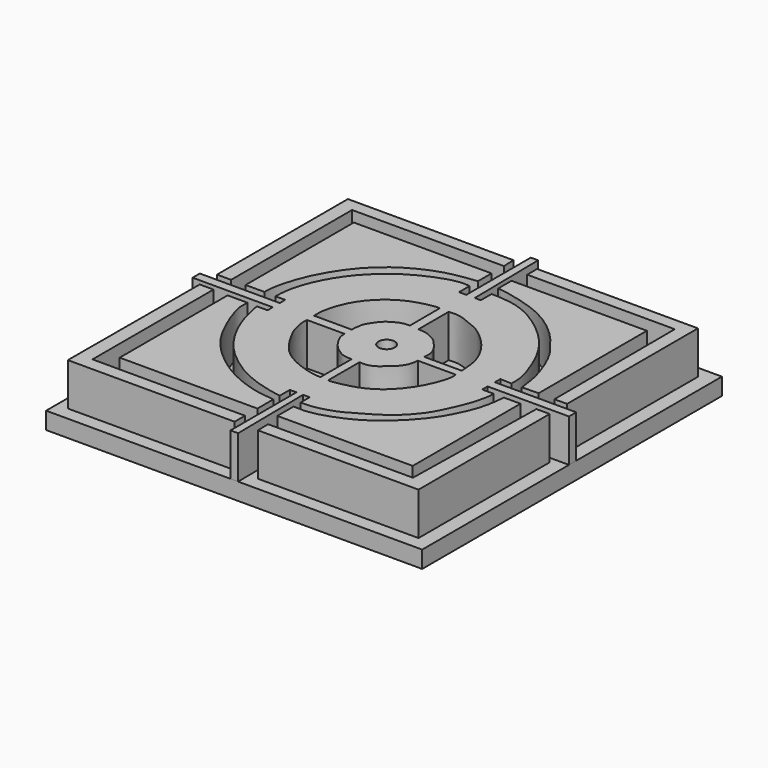
from build123d import *

# Parameters (mm, degrees)
F1_DEPTH = 5
F0_R     = 0.9585003227
F3_DEPTH = 2


# Not quite as in the source:
# - a feature names something its author has since deleted; it is built from what else it names


with BuildPart() as f1:
    # F0 (on Top) → F1 (new body)
    with BuildSketch(Plane.XY):
        with BuildLine():
            add(Edge.make_bspline(
                [(16.4221860468, 62.1270276606), (15.8832675467, 62.1270276606), (15.3443490465, 62.1270276606), (14.8054305464, 62.1270276606)],
                knots=[0, 0, 0, 0, 1.6167555004, 1.6167555004, 1.6167555004, 1.6167555004], degree=3))
            add(Edge.make_bspline(
                [(14.8054305464, 62.1270276606), (14.7858333463, 55.7044409215), (14.7662361463, 49.2818541825), (14.7466389462, 42.8592674434)],
                knots=[0, 0, 0, 0, 19.2678499122, 19.2678499122, 19.2678499122, 19.2678499122], degree=3))
            add(Edge.make_bspline(
                [(14.7466389462, 42.8592674434), (21.2821072588, 42.8592674434), (27.7793089098, 42.8592674434), (34.3147772225, 42.8592674434)],
                knots=[0, 0, 0, 0, 19.5681382762, 19.5681382762, 19.5681382762, 19.5681382762], degree=3))
            add(Edge.make_bspline(
                [(34.3147772225, 42.8592674434), (34.3147772225, 43.3677670856), (34.3147772225, 43.8762667278), (34.3147772225, 44.3847663701)],
                knots=[0, 0, 0, 0, 1.5254989266, 1.5254989266, 1.5254989266, 1.5254989266], degree=3))
            add(Edge.make_bspline(
                [(34.3147772225, 44.3847663701), (28.3378246101, 44.3847663701), (22.3991386592, 44.3847663701), (16.4221860468, 44.3847663701)],
                knots=[0, 0, 0, 0, 17.8925911756, 17.8925911756, 17.8925911756, 17.8925911756], degree=3))
            add(Edge.make_bspline(
                [(16.4221860468, 44.3847663701), (16.4221860468, 50.2988534669), (16.4221860468, 56.2129405638), (16.4221860468, 62.1270276606)],
                knots=[0, 0, 0, 0, 17.7422612906, 17.7422612906, 17.7422612906, 17.7422612906], degree=3))
        make_face()
    extrude(amount=-F1_DEPTH)


with BuildPart() as f1b:
    # F0 (on Top) → F1, piece 2 (new body)
    with BuildSketch(Plane.XY):
        with BuildLine():
            add(Edge.make_bspline(
                [(54.01673913, 44.3847663701), (48.3487062156, 44.3847663701), (42.6806733012, 44.3847663701), (37.0126403868, 44.3847663701)],
                knots=[0, 0, 0, 0, 17.0040987432, 17.0040987432, 17.0040987432, 17.0040987432], degree=3))
            add(Edge.make_bspline(
                [(37.0126403868, 44.3847663701), (37.0219697555, 43.8762667278), (37.0312991242, 43.3677670856), (37.0406284928, 42.8592674434)],
                knots=[0, 0, 0, 0, 1.5257556519, 1.5257556519, 1.5257556519, 1.5257556519], degree=3))
            add(Edge.make_bspline(
                [(37.0406284928, 42.8592674434), (43.3241464198, 42.8592674434), (49.6076643467, 42.8592674434), (55.8911822736, 42.8592674434)],
                knots=[0, 0, 0, 0, 18.8505537808, 18.8505537808, 18.8505537808, 18.8505537808], degree=3))
            add(Edge.make_bspline(
                [(55.8911822736, 42.8592674434), (55.8911822736, 49.2690689862), (55.8911822736, 55.6788705289), (55.8911822736, 62.0886720717)],
                knots=[0, 0, 0, 0, 19.2294046283, 19.2294046283, 19.2294046283, 19.2294046283], degree=3))
            add(Edge.make_bspline(
                [(55.8911822736, 62.0886720717), (55.3724678854, 62.0886720717), (54.8537534972, 62.0886720717), (54.335039109, 62.0886720717)],
                knots=[0, 0, 0, 0, 1.5561431646, 1.5561431646, 1.5561431646, 1.5561431646], degree=3))
            add(Edge.make_bspline(
                [(54.335039109, 62.0886720717), (54.228939116, 56.1873701711), (54.122839123, 50.2860682706), (54.01673913, 44.3847663701)],
                knots=[0, 0, 0, 0, 17.7067668412, 17.7067668412, 17.7067668412, 17.7067668412], degree=3))
        make_face()
    extrude(amount=-F1_DEPTH)


with BuildPart() as f1c:
    # F0 (on Top) → F1, piece 3 (new body)
    with BuildSketch(Plane.XY):
        with BuildLine():
            add(Edge.make_bspline(
                [(54.335039109, 82.3838636279), (54.3570650948, 76.470060481), (54.3790910807, 70.556257334), (54.4011170665, 64.6424541871)],
                knots=[0, 0, 0, 0, 17.7415324942, 17.7415324942, 17.7415324942, 17.7415324942], degree=3))
            add(Edge.make_bspline(
                [(54.4011170665, 64.6424541871), (54.8964854744, 64.6476306849), (55.3918538822, 64.6528071827), (55.88722229, 64.6579836805)],
                knots=[0, 0, 0, 0, 1.4861863613, 1.4861863613, 1.4861863613, 1.4861863613], degree=3))
            add(Edge.make_bspline(
                [(55.88722229, 64.6579836805), (55.88722229, 71.0520827108), (55.88722229, 77.446181741), (55.88722229, 83.8402807713)],
                knots=[0, 0, 0, 0, 19.1822970907, 19.1822970907, 19.1822970907, 19.1822970907], degree=3))
            add(Edge.make_bspline(
                [(55.88722229, 83.8402807713), (49.5988047785, 83.8402807713), (43.310387267, 83.8402807713), (37.0219697555, 83.8402807713)],
                knots=[0, 0, 0, 0, 18.8652525345, 18.8652525345, 18.8652525345, 18.8652525345], degree=3))
            add(Edge.make_bspline(
                [(37.0219697555, 83.8402807713), (37.0219697555, 83.3548083901), (37.0219697555, 82.869336009), (37.0219697555, 82.3838636279)],
                knots=[0, 0, 0, 0, 1.4564171433, 1.4564171433, 1.4564171433, 1.4564171433], degree=3))
            add(Edge.make_bspline(
                [(37.0219697555, 82.3838636279), (42.7929928733, 82.3838636279), (48.5640159912, 82.3838636279), (54.335039109, 82.3838636279)],
                knots=[0, 0, 0, 0, 17.3130693535, 17.3130693535, 17.3130693535, 17.3130693535], degree=3))
        make_face()
    extrude(amount=-F1_DEPTH)


with BuildPart() as f1d:
    # F0 (on Top) → F1, piece 4 (new body)
    with BuildSketch(Plane.XY):
        with BuildLine():
            add(Edge.make_bspline(
                [(16.4753869176, 82.3838636279), (22.4143899977, 82.3838636279), (28.3533930779, 82.3838636279), (34.292396158, 82.3838636279)],
                knots=[0, 0, 0, 0, 17.8170092404, 17.8170092404, 17.8170092404, 17.8170092404], degree=3))
            add(Edge.make_bspline(
                [(34.292396158, 82.3838636279), (34.2783766488, 82.869336009), (34.2643571397, 83.3548083901), (34.2503376305, 83.8402807713)],
                knots=[0, 0, 0, 0, 1.4570243015, 1.4570243015, 1.4570243015, 1.4570243015], degree=3))
            add(Edge.make_bspline(
                [(34.2503376305, 83.8402807713), (27.7733197436, 83.8402807713), (21.2963018566, 83.8402807713), (14.8192839697, 83.8402807713)],
                knots=[0, 0, 0, 0, 19.4310536608, 19.4310536608, 19.4310536608, 19.4310536608], degree=3))
            add(Edge.make_bspline(
                [(14.8192839697, 83.8402807713), (14.8192839697, 77.4410052432), (14.8192839697, 71.0417297151), (14.8192839697, 64.6424541871)],
                knots=[0, 0, 0, 0, 19.1978265842, 19.1978265842, 19.1978265842, 19.1978265842], degree=3))
            add(Edge.make_bspline(
                [(14.8192839697, 64.6424541871), (15.3713182857, 64.6424541871), (15.9233526016, 64.6424541871), (16.4753869176, 64.6424541871)],
                knots=[0, 0, 0, 0, 1.6561029479, 1.6561029479, 1.6561029479, 1.6561029479], degree=3))
            add(Edge.make_bspline(
                [(16.4753869176, 64.6424541871), (16.4753869176, 70.556257334), (16.4753869176, 76.470060481), (16.4753869176, 82.3838636279)],
                knots=[0, 0, 0, 0, 17.7414094408, 17.7414094408, 17.7414094408, 17.7414094408], degree=3))
        make_face()
    extrude(amount=-F1_DEPTH)


with BuildPart() as f1e:
    # F0 (on Top) → F1, piece 5 (new body)
    with BuildSketch(Plane.XY):
        with BuildLine():
            add(Edge.make_bspline(
                [(34.3147772225, 48.5477223992), (34.3147772225, 47.7679459265), (34.3147772225, 46.988146883), (34.3147772225, 46.2066438408)],
                knots=[2.4039060836, 2.4039060836, 2.4039060836, 2.4039060836, 4.7449614652, 4.7449614652, 4.7449614652, 4.7449614652], degree=3))
            add(Edge.make_bspline(
                [(20.4879599351, 62.0290902522), (20.4693214602, 61.6671803247), (20.4285047326, 60.8746151567), (20.8482271329, 59.3461065055), (22.256354868, 55.8366403204), (24.3117786608, 53.167039142), (26.7550892134, 51.1628748476), (28.919099348, 49.8625881243), (31.7597491149, 48.8010015971), (33.4812459256, 48.6296137105), (34.3147772225, 48.5477223992)],
                knots=[0, 0, 0, 0, 0.081894709, 0.1794303416, 0.3310168589, 0.4773374309, 0.6145674727, 0.7394518428, 0.8745421592, 1, 1, 1, 1], degree=3))
            add(Edge.make_bspline(
                [(20.4879599351, 62.0290902522), (19.6947968911, 62.0290902522), (18.9461487655, 62.0290902522), (18.1529857215, 62.0290902522)],
                knots=[0, 0, 0, 0, 2.3349742136, 2.3349742136, 2.3349742136, 2.3349742136], degree=3))
            add(Edge.make_bspline(
                [(18.1529857215, 62.0290902522), (18.1529857215, 56.7574902045), (18.1529857215, 51.4782438884), (18.1529857215, 46.2066438408)],
                knots=[0, 0, 0, 0, 15.8224464113, 15.8224464113, 15.8224464113, 15.8224464113], degree=3))
            add(Edge.make_bspline(
                [(18.1529857215, 46.2066438408), (23.553005109, 46.2066438408), (28.9147578349, 46.2066438408), (34.3147772225, 46.2066438408)],
                knots=[0, 0, 0, 0, 16.161791501, 16.161791501, 16.161791501, 16.161791501], degree=3))
        make_face()
    extrude(amount=-F1_DEPTH)


with BuildPart() as f1f:
    # F0 (on Top) → F1, piece 6 (new body)
    with BuildSketch(Plane.XY):
        with BuildLine():
            add(Edge.make_bspline(
                [(36.6532574268, 48.5900547715), (37.1659984015, 48.5539380597), (38.3612666094, 48.4722841885), (41.259498319, 49.3013045058), (44.6677584405, 51.0956087564), (47.6122450219, 54.2241767739), (48.8379845975, 56.1122685743), (50.2796461417, 59.1401877289), (50.4957243282, 61.0016312164), (50.5860532031, 62.0105434568)],
                knots=[0, 0, 0, 0, 0.106158071, 0.2479012264, 0.4137983248, 0.5833888307, 0.7094215409, 0.8578219688, 0.9998455807, 0.9998455807, 0.9998455807, 0.9998455807], degree=3))
            add(Edge.make_bspline(
                [(36.6532574268, 48.5900547715), (36.6532574268, 47.796167775), (36.6532574268, 47.0022889217), (36.6532574268, 46.2066438408)],
                knots=[2.3615424662, 2.3615424662, 2.3615424662, 2.3615424662, 4.7449614652, 4.7449614652, 4.7449614652, 4.7449614652], degree=3))
            add(Edge.make_bspline(
                [(36.6532574268, 46.2066438408), (41.9390395454, 46.2066438408), (47.2448796724, 46.2066438408), (52.530661791, 46.2066438408)],
                knots=[0, 0, 0, 0, 15.8774043642, 15.8774043642, 15.8774043642, 15.8774043642], degree=3))
            add(Edge.make_bspline(
                [(52.530661791, 46.2066438408), (52.530661791, 51.4746103795), (52.530661791, 56.7425769182), (52.530661791, 62.0105434568)],
                knots=[0, 0, 0, 0, 15.803899616, 15.803899616, 15.803899616, 15.803899616], degree=3))
            add(Edge.make_bspline(
                [(52.530661791, 62.0105434568), (51.8768814433, 62.0096531905), (51.2359389259, 62.0064264969), (50.5860532031, 62.0105434568)],
                knots=[0, 0, 0, 0, 1.944608588, 1.944608588, 1.944608588, 1.944608588], degree=3))
        make_face()
    extrude(amount=-F1_DEPTH)


with BuildPart() as f1g:
    # F0 (on Top) → F1, piece 7 (new body)
    with BuildSketch(Plane.XY):
        with BuildLine():
            add(Edge.make_bspline(
                [(50.586347787, 64.6269246936), (50.4902843865, 65.4274965576), (50.3599208327, 67.1057626927), (48.9639078696, 70.7124599907), (48.1054743858, 71.9302188038), (47.5525483489, 72.5759938359)],
                knots=[0, 0, 0, 0, 0.3131338762, 0.6947785119, 1, 1, 1, 1], degree=3))
            add(Edge.make_bspline(
                [(52.530661791, 64.673513174), (51.8854191596, 64.6579836805), (51.2315904185, 64.6424541871), (50.586347787, 64.6269246936)],
                knots=[0, 0, 0, 0, 1.9448720865, 1.9448720865, 1.9448720865, 1.9448720865], degree=3))
            add(Edge.make_bspline(
                [(52.530661791, 64.673513174), (52.530661791, 69.9629137913), (52.530661791, 75.2523144086), (52.530661791, 80.5417150259)],
                knots=[0, 0, 0, 0, 15.8682018518, 15.8682018518, 15.8682018518, 15.8682018518], degree=3))
            add(Edge.make_bspline(
                [(52.530661791, 80.5417150259), (47.2448796724, 80.5417150259), (41.9390395454, 80.5417150259), (36.6532574268, 80.5417150259)],
                knots=[0, 0, 0, 0, 15.8774043642, 15.8774043642, 15.8774043642, 15.8774043642], degree=3))
            add(Edge.make_bspline(
                [(36.6532574268, 80.5417150259), (36.6532574268, 79.8772449294), (36.6532574268, 79.212774833), (36.6532574268, 78.5483047366)],
                knots=[0, 0, 0, 0, 1.9934102893, 1.9934102893, 1.9934102893, 1.9934102893], degree=3))
            add(Edge.make_bspline(
                [(36.6532574268, 78.5483047366), (36.7126410377, 78.5483047366), (36.8102913102, 78.5483047366), (36.869674921, 78.5483047366)],
                knots=[0, 0, 0, 0, 0.2164174942, 0.2164174942, 0.2164174942, 0.2164174942], degree=3))
            add(Edge.make_bspline(
                [(47.5525483489, 72.5759938359), (47.2094456379, 73.0452450886), (46.3251874314, 74.2546184271), (42.8264679604, 77.3738653562), (37.7096081399, 78.4877127771), (37.0498966569, 78.5353037172), (36.869674921, 78.5483047366)],
                knots=[0, 0, 0, 0, 0.2081289099, 0.5363982582, 0.8733520443, 1, 1, 1, 1], degree=3))
        make_face()
    extrude(amount=-F1_DEPTH)


with BuildPart() as f1h:
    # F0 (on Top) → F1, piece 8 (new body)
    with BuildSketch(Plane.XY):
        with BuildLine():
            add(Edge.make_bspline(
                [(20.3758893793, 64.673513174), (20.361082674, 64.8867621856), (20.3251453414, 65.5485311624), (20.9459669611, 68.3899563783), (22.6616462733, 71.9773117462), (25.7168833882, 75.7093585738), (30.4989234722, 78.1408190427), (33.1097507297, 78.4201280734), (34.3078970909, 78.5483047366)],
                knots=[0.0055230612, 0.0055230612, 0.0055230612, 0.0055230612, 0.0812499649, 0.2333418136, 0.4167906579, 0.6159670421, 0.8237651507, 1, 1, 1, 1], degree=3))
            add(Edge.make_bspline(
                [(34.3078970909, 80.5417150259), (34.3078970909, 79.8772449294), (34.3078970909, 79.212774833), (34.3078970909, 78.5483047366)],
                knots=[0, 0, 0, 0, 1.9934102893, 1.9934102893, 1.9934102893, 1.9934102893], degree=3))
            add(Edge.make_bspline(
                [(34.3078970909, 80.5417150259), (28.9229266346, 80.5417150259), (23.5379561778, 80.5417150259), (18.1529857215, 80.5417150259)],
                knots=[0, 0, 0, 0, 16.1549113694, 16.1549113694, 16.1549113694, 16.1549113694], degree=3))
            add(Edge.make_bspline(
                [(18.1529857215, 80.5417150259), (18.1529857215, 75.2523144086), (18.1529857215, 69.9629137913), (18.1529857215, 64.673513174)],
                knots=[0, 0, 0, 0, 15.8682018518, 15.8682018518, 15.8682018518, 15.8682018518], degree=3))
            add(Edge.make_bspline(
                [(18.1529857215, 64.673513174), (18.8939536091, 64.673513174), (19.6349214917, 64.673513174), (20.3758893793, 64.673513174)],
                knots=[0, 0, 0, 0, 2.2229036578, 2.2229036578, 2.2229036578, 2.2229036578], degree=3))
        make_face()
    extrude(amount=-F1_DEPTH)


with BuildPart() as f1i:
    # F0 (on Top) → F1, piece 9 (new body)
    with BuildSketch(Plane.XY):
        with BuildLine():
            add(Edge.make_bspline(
                [(22.8586476296, 62.7715587616), (19.72528516, 62.7715587616), (16.5919226905, 62.7715587616), (13.4585602209, 62.7715587616)],
                knots=[0, 0, 0, 0, 9.4000874087, 9.4000874087, 9.4000874087, 9.4000874087], degree=3))
            add(Edge.make_bspline(
                [(22.8376183659, 63.8296038931), (22.8446281205, 63.4721076514), (22.851637875, 63.1290550033), (22.8586476296, 62.7715587616)],
                knots=[0, 0, 0, 0, 1.0582540953, 1.0582540953, 1.0582540953, 1.0582540953], degree=3))
            add(Edge.make_bspline(
                [(13.4585602209, 63.8296038931), (16.5849129359, 63.8296038931), (19.7112656509, 63.8296038931), (22.8376183659, 63.8296038931)],
                knots=[0, 0, 0, 0, 9.379058145, 9.379058145, 9.379058145, 9.379058145], degree=3))
            add(Edge.make_bspline(
                [(13.4585602209, 62.7715587616), (13.4585602209, 63.1290550033), (13.4585602209, 63.4721076514), (13.4585602209, 63.8296038931)],
                knots=[0, 0, 0, 0, 1.0580451315, 1.0580451315, 1.0580451315, 1.0580451315], degree=3))
        make_face()
        with BuildLine():
            add(Edge.make_bspline(
                [(35.1613126695, 85.2358043194), (35.1614827911, 82.0812707146), (35.1616529127, 78.9267371098), (35.1618230343, 75.772203505)],
                knots=[0, 0, 0, 0, 9.4636008281, 9.4636008281, 9.4636008281, 9.4636008281], degree=3))
            add(Edge.make_bspline(
                [(36.1621901393, 75.772203505), (35.8287344376, 75.772203505), (35.495278736, 75.772203505), (35.1618230343, 75.772203505)],
                knots=[0.7074847817, 0.7074847817, 0.7074847817, 0.7074847817, 1.7078518867, 1.7078518867, 1.7078518867, 1.7078518867], degree=3))
            add(Edge.make_bspline(
                [(36.1621901393, 75.772203505), (36.1133764187, 78.9267371098), (36.0645626982, 82.0812707146), (36.0157489777, 85.2358043194)],
                knots=[0, 0, 0, 0, 9.4647337726, 9.4647337726, 9.4647337726, 9.4647337726], degree=3))
            add(Edge.make_bspline(
                [(36.0157489777, 85.2358043194), (35.7309368749, 85.2358043194), (35.4461247722, 85.2358043194), (35.1613126695, 85.2358043194)],
                knots=[0, 0, 0, 0, 0.8544363081, 0.8544363081, 0.8544363081, 0.8544363081], degree=3))
        make_face()
        with BuildLine():
            add(Edge.make_bspline(
                [(48.0358153582, 62.8075450659), (48.0358153582, 63.1565873665), (48.0358153582, 63.5197117493), (48.0358153582, 63.8690404594)],
                knots=[0.8139980546, 0.8139980546, 0.8139980546, 0.8139980546, 1.8351889303, 1.8351889303, 1.8351889303, 1.8351889303], degree=3))
            add(Edge.make_bspline(
                [(57.5837679207, 62.8075450659), (54.4011170665, 62.8075450659), (51.2184662124, 62.8075450659), (48.0358153582, 62.8075450659)],
                knots=[0, 0, 0, 0, 9.5479525626, 9.5479525626, 9.5479525626, 9.5479525626], degree=3))
            add(Edge.make_bspline(
                [(57.5837679207, 63.8690404594), (57.5837679207, 63.5152086615), (57.5837679207, 63.1613768637), (57.5837679207, 62.8075450659)],
                knots=[0, 0, 0, 0, 1.0614953935, 1.0614953935, 1.0614953935, 1.0614953935], degree=3))
            add(Edge.make_bspline(
                [(48.0358153582, 63.8690404594), (51.2184662124, 63.8690404594), (54.4011170665, 63.8690404594), (57.5837679207, 63.8690404594)],
                knots=[0, 0, 0, 0, 9.5479525626, 9.5479525626, 9.5479525626, 9.5479525626], degree=3))
        make_face()
        with BuildLine():
            add(Edge.make_bspline(
                [(34.3147772225, 50.9516053061), (34.3147772225, 50.4543464832), (34.3147772225, 49.9577775393), (34.3147772225, 49.4614653289)],
                knots=[0, 0, 0, 0, 1.4895789018, 1.4895789018, 1.4895789018, 1.4895789018], degree=3))
            add(Edge.make_bspline(
                [(34.3147772225, 50.9516053061), (34.5746083563, 50.9516053061), (34.8344394901, 50.9516053061), (35.0942706239, 50.9516053061)],
                knots=[0, 0, 0, 0, 0.7794934014, 0.7794934014, 0.7794934014, 0.7794934014], degree=3))
            add(Edge.make_bspline(
                [(35.0942706239, 50.9516053061), (35.3541017577, 50.9516053061), (35.6139328915, 50.9516053061), (35.8737640253, 50.9516053061)],
                knots=[0.7794934014, 0.7794934014, 0.7794934014, 0.7794934014, 1.5589868029, 1.5589868029, 1.5589868029, 1.5589868029], degree=3))
            add(Edge.make_bspline(
                [(35.8737640253, 50.9516053061), (36.1335951592, 50.9516053061), (36.393426293, 50.9516053061), (36.6532574268, 50.9516053061)],
                knots=[1.5589868029, 1.5589868029, 1.5589868029, 1.5589868029, 2.3384802043, 2.3384802043, 2.3384802043, 2.3384802043], degree=3))
            add(Edge.make_bspline(
                [(36.6532574268, 50.9516053061), (36.6532574268, 50.505140304), (36.6532574268, 50.0592314401), (36.6532574268, 49.6135652065)],
                knots=[0, 0, 0, 0, 1.3374219158, 1.3374219158, 1.3374219158, 1.3374219158], degree=3))
            add(Edge.make_bspline(
                [(49.3640676141, 62.0138347149), (49.3773776963, 61.8140856389), (49.4091537047, 61.4383259718), (48.9438098259, 59.271970581), (47.9323980402, 57.0865478886), (47.0309852149, 55.1649399571), (44.7426629609, 52.6459886677), (41.9053558743, 51.1477208977), (40.6474280883, 50.3668186777), (38.3658464203, 49.6107956621), (37.1929678959, 49.6135527756), (36.6532574268, 49.6135652065)],
                knots=[0, 0, 0, 0, 0.0578187886, 0.1702588875, 0.2925946382, 0.4048109482, 0.5478243019, 0.6853752174, 0.7807855987, 0.8983940872, 1, 1, 1, 1], degree=3))
            add(Edge.make_bspline(
                [(49.3640676141, 62.0138347149), (48.9213168621, 62.0138347149), (48.4785661101, 62.0138347149), (48.0358153582, 62.0138347149)],
                knots=[0, 0, 0, 0, 1.3282522559, 1.3282522559, 1.3282522559, 1.3282522559], degree=3))
            add(Edge.make_bspline(
                [(48.0358153582, 62.0138347149), (48.0358153582, 62.2600446364), (48.0358153582, 62.5293211212), (48.0358153582, 62.8075450659)],
                knots=[0, 0, 0, 0, 0.8139980546, 0.8139980546, 0.8139980546, 0.8139980546], degree=3))
            add(Edge.make_bspline(
                [(48.0358153582, 62.8075450659), (48.0358153582, 63.1565873665), (48.0358153582, 63.5197117493), (48.0358153582, 63.8690404594)],
                knots=[0.8139980546, 0.8139980546, 0.8139980546, 0.8139980546, 1.8351889303, 1.8351889303, 1.8351889303, 1.8351889303], degree=3))
            add(Edge.make_bspline(
                [(48.0358153582, 63.8690404594), (48.0358153582, 64.1510816237), (48.0358153582, 64.4241298972), (48.0358153582, 64.673513174)],
                knots=[1.8351889303, 1.8351889303, 1.8351889303, 1.8351889303, 2.6596784591, 2.6596784591, 2.6596784591, 2.6596784591], degree=3))
            add(Edge.make_bspline(
                [(48.0358153582, 64.673513174), (48.4824304779, 64.6579836806), (48.9290455977, 64.6424541871), (49.3756607175, 64.6269246936)],
                knots=[0, 0, 0, 0, 1.3406550911, 1.3406550911, 1.3406550911, 1.3406550911], degree=3))
            add(Edge.make_bspline(
                [(36.869674921, 77.3325264454), (37.0804886913, 77.3451733979), (37.6488734826, 77.350612493), (39.857399112, 77.1542788889), (42.0612404884, 76.2032987688), (44.3444346233, 74.6008118443), (46.336657962, 72.6531262304), (47.7950787284, 70.3663611306), (48.7349733481, 68.1317289371), (49.4042837293, 66.0976157093), (49.3845737131, 65.084903481), (49.3756607175, 64.6269246936)],
                knots=[0, 0, 0, 0, 0.0654086489, 0.1773681339, 0.2974935373, 0.4246372311, 0.5524322165, 0.6778681778, 0.7977350761, 0.9086148136, 1, 1, 1, 1], degree=3))
            add(Edge.make_bspline(
                [(36.869674921, 77.3325264454), (36.869674921, 76.768271625), (36.869674921, 76.3364583254), (36.869674921, 75.772203505)],
                knots=[0, 0, 0, 0, 1.5603229403, 1.5603229403, 1.5603229403, 1.5603229403], degree=3))
            add(Edge.make_bspline(
                [(36.869674921, 75.772203505), (36.6338466605, 75.772203505), (36.3980183999, 75.772203505), (36.1621901393, 75.772203505)],
                knots=[0, 0, 0, 0, 0.7074847817, 0.7074847817, 0.7074847817, 0.7074847817], degree=3))
            add(Edge.make_bspline(
                [(36.1621901393, 75.772203505), (35.8287344376, 75.772203505), (35.495278736, 75.772203505), (35.1618230343, 75.772203505)],
                knots=[0.7074847817, 0.7074847817, 0.7074847817, 0.7074847817, 1.7078518867, 1.7078518867, 1.7078518867, 1.7078518867], degree=3))
            add(Edge.make_bspline(
                [(35.1618230343, 75.772203505), (34.8771810532, 75.772203505), (34.592539072, 75.772203505), (34.3078970909, 75.772203505)],
                knots=[1.7078518867, 1.7078518867, 1.7078518867, 1.7078518867, 2.5617778301, 2.5617778301, 2.5617778301, 2.5617778301], degree=3))
            add(Edge.make_bspline(
                [(34.3078970909, 75.772203505), (34.3078970909, 76.3364583254), (34.3078970909, 76.768271625), (34.3078970909, 77.3325264454)],
                knots=[0, 0, 0, 0, 1.5603229403, 1.5603229403, 1.5603229403, 1.5603229403], degree=3))
            add(Edge.make_bspline(
                [(34.3078970909, 77.3325264454), (33.8691194926, 77.382322327), (32.8361100051, 77.4689395129), (29.8155548786, 76.4208925059), (27.0907434314, 74.7925930891), (24.3723664588, 72.2446092205), (22.390718826, 68.7672813299), (21.7368975728, 66.1289348712), (21.7024073564, 65.0743365342), (21.6877348721, 64.6269246936)],
                knots=[0, 0, 0, 0, 0.1030970948, 0.2558297354, 0.4125735671, 0.5797448281, 0.7543120874, 0.896055567, 1, 1, 1, 1], degree=3))
            add(Edge.make_bspline(
                [(21.6877348721, 64.6269246936), (22.07102937, 64.6269246936), (22.454323868, 64.6269246936), (22.8376183659, 64.6269246936)],
                knots=[0, 0, 0, 0, 1.1498834938, 1.1498834938, 1.1498834938, 1.1498834938], degree=3))
            add(Edge.make_bspline(
                [(22.8376183659, 64.6269246936), (22.8376183659, 64.3659656247), (22.8376183659, 64.0905629621), (22.8376183659, 63.8296038931)],
                knots=[0, 0, 0, 0, 0.7973208005, 0.7973208005, 0.7973208005, 0.7973208005], degree=3))
            add(Edge.make_bspline(
                [(22.8376183659, 63.8296038931), (22.8446281205, 63.4721076514), (22.851637875, 63.1290550033), (22.8586476296, 62.7715587616)],
                knots=[0, 0, 0, 0, 1.0582540953, 1.0582540953, 1.0582540953, 1.0582540953], degree=3))
            add(Edge.make_bspline(
                [(22.8586476296, 62.7715587616), (22.8586476296, 62.5182241201), (22.8586476296, 62.2638780983), (22.8586476296, 62.0105434568)],
                knots=[0, 0, 0, 0, 0.7610153048, 0.7610153048, 0.7610153048, 0.7610153048], degree=3))
            add(Edge.make_bspline(
                [(22.8586476296, 62.0105434568), (22.4407364925, 62.0067709795), (22.0190702627, 62.0035008976), (21.6011591256, 61.9997284202)],
                knots=[0, 0, 0, 0, 1.2575350106, 1.2575350106, 1.2575350106, 1.2575350106], degree=3))
            add(Edge.make_bspline(
                [(34.3147772225, 49.4614653289), (33.9245960474, 49.5285893774), (33.0861653986, 49.6843381279), (30.8988287416, 50.2399232722), (28.7037531402, 51.2397646623), (26.701560584, 52.6385865663), (24.7154817236, 54.4489638152), (23.2796660294, 56.7950585788), (22.6355857925, 58.2054167119), (22.031128361, 59.8270974156), (21.6139264874, 61.9657285373), (21.6011591256, 61.9997284202)],
                knots=[0, 0, 0, 0, 0.0839435245, 0.1971299906, 0.3159478434, 0.4339870618, 0.5595316455, 0.6844601215, 0.7770486709, 0.8847753942, 0.9909823169, 0.9909823169, 0.9909823169, 0.9909823169], degree=3))
        make_face()
        with BuildLine():
            add(Edge.make_bspline(
                [(34.925326705, 52.603892982), (35.2390151885, 52.603892982), (35.5600755418, 52.603892982), (35.8737640253, 52.603892982)],
                knots=[0, 0, 0, 0, 0.9484373204, 0.9484373204, 0.9484373204, 0.9484373204], degree=3))
            add(Edge.make_bspline(
                [(34.925326705, 52.603892982), (34.925326705, 53.2904155552), (34.925326705, 53.9769381285), (34.925326705, 54.6634607017)],
                knots=[0, 0, 0, 0, 2.0595677197, 2.0595677197, 2.0595677197, 2.0595677197], degree=3))
            add(Edge.make_bspline(
                [(34.925326705, 54.6634607017), (34.5518732178, 54.6953086569), (33.717308623, 54.7664811298), (31.9803682635, 55.3030649205), (30.0705372898, 56.2301299661), (28.5641309525, 57.8363424843), (27.30750677, 60.1032276072), (27.0857106902, 60.9224580546), (26.8248005822, 61.9684883134), (26.8571916762, 62.5073209315), (26.8724666288, 62.7632349485)],
                knots=[0, 0, 0, 0, 0.110767808, 0.2477353648, 0.3952208787, 0.5492551845, 0.7107905198, 0.8058986774, 0.9089425501, 1, 1, 1, 1], degree=3))
            add(Edge.make_bspline(
                [(26.8724666288, 62.7632349485), (26.1553658275, 62.7632349485), (25.4382281575, 62.7632349485), (24.7209798545, 62.7632349485)],
                knots=[4.3020518153, 4.3020518153, 4.3020518153, 4.3020518153, 6.4534648652, 6.4534648652, 6.4534648652, 6.4534648652], degree=3))
            add(Edge.make_bspline(
                [(24.7209798545, 62.7632349485), (24.7209798545, 63.1207311902), (24.7209798545, 63.4721076514), (24.7209798545, 63.8296038931)],
                knots=[0, 0, 0, 0, 1.0663689446, 1.0663689446, 1.0663689446, 1.0663689446], degree=3))
            add(Edge.make_bspline(
                [(24.7209798545, 63.8296038931), (25.4382281575, 63.8296038931), (26.1553658275, 63.8296038931), (26.8724666288, 63.8296038931)],
                knots=[0, 0, 0, 0, 2.15141305, 2.15141305, 2.15141305, 2.15141305], degree=3))
            add(Edge.make_bspline(
                [(26.8724666288, 63.8296038931), (26.8499961986, 64.1297128203), (26.7915511509, 64.9159854796), (27.4489442843, 67.5424528115), (29.1460281439, 69.8668946254), (31.2630920945, 71.3711755056), (33.089488459, 71.9498298458), (34.5543238979, 72.2526141567), (34.8216077873, 72.167279821), (34.9269575947, 72.1403943419)],
                knots=[0, 0, 0, 0, 0.1107865405, 0.2883106705, 0.4762985602, 0.6506645751, 0.8052278461, 0.9348910644, 0.9981834356, 0.9981834356, 0.9981834356, 0.9981834356], degree=3))
            add(Edge.make_bspline(
                [(34.9269575963, 72.1403943453), (34.9322233756, 72.8452225471), (34.9376056923, 73.5426126165), (34.9383429328, 74.2186774767)],
                knots=[4.3493758064, 4.3493758064, 4.3493758064, 4.3493758064, 6.4429306287, 6.4429306287, 6.4429306287, 6.4429306287], degree=3))
            add(Edge.make_bspline(
                [(34.9383429328, 74.2186774767), (35.2495996295, 74.2186774767), (35.6934691469, 74.2186774767), (36.0047258437, 74.2186774767)],
                knots=[0, 0, 0, 0, 1.0663829109, 1.0663829109, 1.0663829109, 1.0663829109], degree=3))
            add(Edge.make_bspline(
                [(36.0047258437, 74.2186774767), (36.0047258437, 73.5254182137), (36.0047258437, 72.8318119443), (36.0047258437, 72.1380828115)],
                knots=[0, 0, 0, 0, 2.0808522229, 2.0808522229, 2.0808522229, 2.0808522229], degree=3))
            add(Edge.make_bspline(
                [(36.0047258437, 72.1380828115), (36.3938925786, 72.176645341), (37.1892624653, 72.2599562962), (38.9757163438, 71.5218380741), (40.335860763, 70.9495479182), (42.0195417697, 69.445085577), (43.1087909344, 68.0744773396), (44.0926901407, 66.124842047), (44.1822400572, 64.3513256736), (44.230692864, 63.9170887839), (44.2483052611, 63.7592226267)],
                knots=[0, 0, 0, 0, 0.1077744245, 0.2432758717, 0.3669968831, 0.5137362181, 0.6474276726, 0.7949429999, 0.9260083891, 1, 1, 1, 1], degree=3))
            add(Edge.make_bspline(
                [(44.2483052611, 63.7592226267), (44.9148333595, 63.7592226267), (45.5821774024, 63.7592226267), (46.2516993284, 63.7592226267)],
                knots=[4.399939049, 4.399939049, 4.399939049, 4.399939049, 6.4015394985, 6.4015394985, 6.4015394985, 6.4015394985], degree=3))
            add(Edge.make_bspline(
                [(46.2516993284, 63.7592226267), (46.2516993284, 63.4419967731), (46.2516993284, 63.1247709195), (46.2516993284, 62.8075450659)],
                knots=[0, 0, 0, 0, 0.9516775608, 0.9516775608, 0.9516775608, 0.9516775608], degree=3))
            add(Edge.make_bspline(
                [(46.2516993284, 62.8075450659), (45.6021366131, 62.8075450659), (44.9546238661, 62.8075450659), (44.3079173565, 62.8075450659)],
                knots=[0, 0, 0, 0, 1.9419304618, 1.9419304618, 1.9419304618, 1.9419304618], degree=3))
            add(Edge.make_bspline(
                [(44.3079173565, 62.8075450659), (44.3283324966, 62.5892448609), (44.3809451632, 62.0261342811), (43.8079385586, 60.2268256881), (42.9510376987, 58.6122561047), (41.5549357563, 56.761461728), (39.356308551, 55.1800743795), (36.5251655082, 54.635368342), (36.0075486841, 54.5833842133), (35.8708444479, 54.6613494837)],
                knots=[0, 0, 0, 0, 0.093482767, 0.240545887, 0.3901118201, 0.5529985864, 0.7355469128, 0.9178153363, 0.9992725913, 0.9992725913, 0.9992725913, 0.9992725913], degree=3))
            add(Edge.make_bspline(
                [(35.8737640253, 52.603892982), (35.8716559757, 53.2640846854), (35.8708993911, 53.9547948475), (35.8708444561, 54.6613494909)],
                knots=[0, 0, 0, 0, 2.1233855209, 2.1233855209, 2.1233855209, 2.1233855209], degree=3))
        make_face(mode=Mode.SUBTRACT)
        with BuildLine():
            add(Edge.make_bspline(
                [(34.925326705, 52.603892982), (34.925326705, 53.2904155552), (34.925326705, 53.9769381285), (34.925326705, 54.6634607017)],
                knots=[0, 0, 0, 0, 2.0595677197, 2.0595677197, 2.0595677197, 2.0595677197], degree=3))
            add(Edge.make_bspline(
                [(34.925326705, 52.603892982), (35.2390151885, 52.603892982), (35.5600755418, 52.603892982), (35.8737640253, 52.603892982)],
                knots=[0, 0, 0, 0, 0.9484373204, 0.9484373204, 0.9484373204, 0.9484373204], degree=3))
            add(Edge.make_bspline(
                [(35.8737640253, 52.603892982), (35.8716559757, 53.2640846854), (35.8708993911, 53.9547948475), (35.8708444561, 54.6613494909)],
                knots=[0, 0, 0, 0, 2.1233855209, 2.1233855209, 2.1233855209, 2.1233855209], degree=3))
            add(Edge.make_bspline(
                [(35.8708444561, 54.6613494909), (35.8707280129, 56.15899876), (35.8737640253, 57.7278360235), (35.8737640253, 59.2281147838)],
                knots=[2.1233855209, 2.1233855209, 2.1233855209, 2.1233855209, 6.6242218018, 6.6242218018, 6.6242218018, 6.6242218018], degree=3))
            add(Edge.make_bspline(
                [(35.8737640253, 59.2281147838), (36.1375986032, 59.206205503), (36.7075163857, 59.1593206471), (37.6790674042, 59.5499299549), (38.5039241604, 60.3494299482), (39.1339393314, 60.847880437), (39.6508982285, 61.6650596883), (39.7944701957, 62.2724573743), (39.8429497251, 62.634157849), (39.85015983, 62.8075450659)],
                knots=[0, 0, 0, 0, 0.1415745452, 0.3004976202, 0.4679172727, 0.6103486412, 0.7620373906, 0.8862008469, 1, 1, 1, 1], degree=3))
            add(Edge.make_bspline(
                [(44.3079173565, 62.8075450659), (42.8227672695, 62.8075450659), (41.341869143, 62.8075450659), (39.85015983, 62.8075450659)],
                knots=[1.9419304618, 1.9419304618, 1.9419304618, 1.9419304618, 6.4015394985, 6.4015394985, 6.4015394985, 6.4015394985], degree=3))
            add(Edge.make_bspline(
                [(46.2516993284, 62.8075450659), (45.6021366131, 62.8075450659), (44.9546238661, 62.8075450659), (44.3079173565, 62.8075450659)],
                knots=[0, 0, 0, 0, 1.9419304618, 1.9419304618, 1.9419304618, 1.9419304618], degree=3))
            add(Edge.make_bspline(
                [(46.2516993284, 63.7592226267), (46.2516993284, 63.4419967731), (46.2516993284, 63.1247709195), (46.2516993284, 62.8075450659)],
                knots=[0, 0, 0, 0, 0.9516775608, 0.9516775608, 0.9516775608, 0.9516775608], degree=3))
            add(Edge.make_bspline(
                [(44.2483052611, 63.7592226267), (44.9148333595, 63.7592226267), (45.5821774024, 63.7592226267), (46.2516993284, 63.7592226267)],
                knots=[4.399939049, 4.399939049, 4.399939049, 4.399939049, 6.4015394985, 6.4015394985, 6.4015394985, 6.4015394985], degree=3))
            add(Edge.make_bspline(
                [(39.85015983, 63.7592226267), (41.3219099323, 63.7592226267), (42.783136222, 63.7592226267), (44.2483052611, 63.7592226267)],
                knots=[0, 0, 0, 0, 4.399939049, 4.399939049, 4.399939049, 4.399939049], degree=3))
            add(Edge.make_bspline(
                [(39.85015983, 63.7592226267), (39.8777976251, 64.0737447273), (39.9329895103, 64.7017935092), (39.4930600048, 65.6483420149), (38.7687711469, 66.4902811227), (38.2169656361, 67.0810694819), (37.3194701875, 67.4754133933), (36.8788386257, 67.6308745389), (36.244616478, 67.6874976786), (35.984564616, 67.7026102107), (35.9977702606, 67.7397282926), (36.0047258437, 67.775746848)],
                knots=[0, 0, 0, 0, 0.1354539231, 0.2775958858, 0.425361879, 0.5537700863, 0.6896642415, 0.7891064407, 0.9021048628, 0.9660375021, 1, 1, 1, 1], degree=3))
            add(Edge.make_bspline(
                [(36.0047258437, 72.1380828115), (36.0047258437, 70.6838224675), (36.0047258437, 69.2290222067), (36.0047258437, 67.775746848)],
                knots=[2.0808522229, 2.0808522229, 2.0808522229, 2.0808522229, 6.4429306287, 6.4429306287, 6.4429306287, 6.4429306287], degree=3))
            add(Edge.make_bspline(
                [(36.0047258437, 74.2186774767), (36.0047258437, 73.5254182137), (36.0047258437, 72.8318119443), (36.0047258437, 72.1380828115)],
                knots=[0, 0, 0, 0, 2.0808522229, 2.0808522229, 2.0808522229, 2.0808522229], degree=3))
            add(Edge.make_bspline(
                [(34.9383429328, 74.2186774767), (35.2495996295, 74.2186774767), (35.6934691469, 74.2186774767), (36.0047258437, 74.2186774767)],
                knots=[0, 0, 0, 0, 1.0663829109, 1.0663829109, 1.0663829109, 1.0663829109], degree=3))
            add(Edge.make_bspline(
                [(34.9269575963, 72.1403943453), (34.9322233756, 72.8452225471), (34.9376056923, 73.5426126165), (34.9383429328, 74.2186774767)],
                knots=[4.3493758064, 4.3493758064, 4.3493758064, 4.3493758064, 6.4429306287, 6.4429306287, 6.4429306287, 6.4429306287], degree=3))
            add(Edge.make_bspline(
                [(34.9383429328, 67.775746848), (34.9055811844, 69.179719363), (34.9160179005, 70.6761084827), (34.9269575963, 72.1403943453)],
                knots=[0, 0, 0, 0, 4.3493758064, 4.3493758064, 4.3493758064, 4.3493758064], degree=3))
            add(Edge.make_bspline(
                [(31.3840545714, 64.84041363), (31.4025801674, 64.9870334255), (31.4468089366, 65.3370436448), (31.9660147392, 66.1213993833), (32.5473566892, 66.9601693125), (33.4864505334, 67.4806366522), (33.8671406248, 67.6377467382), (34.4145295536, 67.7949239688), (34.7649020536, 67.7626079202), (34.9383429328, 67.775746848)],
                knots=[0, 0, 0, 0, 0.1186337132, 0.2833790593, 0.4620420695, 0.6363298364, 0.7480335738, 0.8746257605, 1, 1, 1, 1], degree=3))
            add(Edge.make_bspline(
                [(31.287039105, 64.2827898264), (31.3193775938, 64.4686644276), (31.3517160826, 64.6545390288), (31.3840545714, 64.84041363)],
                knots=[0, 0, 0, 0, 0.5660002713, 0.5660002713, 0.5660002713, 0.5660002713], degree=3))
            add(Edge.make_bspline(
                [(31.287039105, 64.0551894903), (31.287039105, 64.131056269), (31.287039105, 64.2069230477), (31.287039105, 64.2827898264)],
                knots=[0, 0, 0, 0, 0.2276003361, 0.2276003361, 0.2276003361, 0.2276003361], degree=3))
            add(Edge.make_bspline(
                [(31.287039105, 63.8296038931), (31.287039105, 63.9024260619), (31.287039105, 64.0093632809), (31.287039105, 64.0441059151), (31.287039105, 64.0551894903)],
                knots=[0, 0, 0, 0, 0.6809805732, 1, 1, 1, 1], degree=3))
            add(Edge.make_bspline(
                [(31.287039105, 63.8296038931), (31.2495076432, 63.8296038931), (31.2119761815, 63.8296038931), (31.1744447197, 63.8296038931)],
                knots=[0, 0, 0, 0, 0.1125943853, 0.1125943853, 0.1125943853, 0.1125943853], degree=3))
            add(Edge.make_bspline(
                [(26.8724666288, 63.8296038931), (28.3064101496, 63.8296038931), (29.7402062484, 63.8296038931), (31.1744447197, 63.8296038931)],
                knots=[2.15141305, 2.15141305, 2.15141305, 2.15141305, 6.4534648652, 6.4534648652, 6.4534648652, 6.4534648652], degree=3))
            add(Edge.make_bspline(
                [(24.7209798545, 63.8296038931), (25.4382281575, 63.8296038931), (26.1553658275, 63.8296038931), (26.8724666288, 63.8296038931)],
                knots=[0, 0, 0, 0, 2.15141305, 2.15141305, 2.15141305, 2.15141305], degree=3))
            add(Edge.make_bspline(
                [(24.7209798545, 62.7632349485), (24.7209798545, 63.1207311902), (24.7209798545, 63.4721076514), (24.7209798545, 63.8296038931)],
                knots=[0, 0, 0, 0, 1.0663689446, 1.0663689446, 1.0663689446, 1.0663689446], degree=3))
            add(Edge.make_bspline(
                [(26.8724666288, 62.7632349485), (26.1553658275, 62.7632349485), (25.4382281575, 62.7632349485), (24.7209798545, 62.7632349485)],
                knots=[4.3020518153, 4.3020518153, 4.3020518153, 4.3020518153, 6.4534648652, 6.4534648652, 6.4534648652, 6.4534648652], degree=3))
            add(Edge.make_bspline(
                [(31.1744447197, 62.7632349485), (29.7402062484, 62.7632349485), (28.3064101496, 62.7632349485), (26.8724666288, 62.7632349485)],
                knots=[0, 0, 0, 0, 4.3020518153, 4.3020518153, 4.3020518153, 4.3020518153], degree=3))
            add(Edge.make_bspline(
                [(31.1744447197, 62.7632349485), (31.211498588, 62.7632349485), (31.2499852367, 62.7632349485), (31.287039105, 62.7632349485)],
                knots=[0, 0, 0, 0, 0.1125943853, 0.1125943853, 0.1125943853, 0.1125943853], degree=3))
            add(Edge.make_bspline(
                [(31.287039105, 62.7632349485), (31.2873385094, 62.5448011128), (31.2881018431, 61.9879022827), (32.2166972547, 60.4273216568), (33.1109275168, 59.7774154203), (33.8040161995, 59.3175506618), (34.5302328639, 59.2596275221), (34.925326705, 59.2281147838)],
                knots=[0, 0, 0, 0, 0.1654329014, 0.4217725195, 0.6261240378, 0.7965950146, 1, 1, 1, 1], degree=3))
            add(Edge.make_bspline(
                [(34.925326705, 54.6634607017), (34.925326705, 56.1850120624), (34.925326705, 57.7065634231), (34.925326705, 59.2281147838)],
                knots=[2.0595677197, 2.0595677197, 2.0595677197, 2.0595677197, 6.6242218018, 6.6242218018, 6.6242218018, 6.6242218018], degree=3))
        make_face()
        with Locations((35.6115102768, 63.5251104832)):
            Circle(F0_R, mode=Mode.SUBTRACT)
        with BuildLine():
            add(Edge.make_bspline(
                [(35.0942706239, 50.9516053061), (35.3541017577, 50.9516053061), (35.6139328915, 50.9516053061), (35.8737640253, 50.9516053061)],
                knots=[0.7794934014, 0.7794934014, 0.7794934014, 0.7794934014, 1.5589868029, 1.5589868029, 1.5589868029, 1.5589868029], degree=3))
            add(Edge.make_bspline(
                [(35.0942706239, 50.9516053061), (35.0942706239, 47.7281509665), (35.0942706239, 44.504696627), (35.0942706239, 41.2812422875)],
                knots=[0, 0, 0, 0, 9.6703630185, 9.6703630185, 9.6703630185, 9.6703630185], degree=3))
            add(Edge.make_bspline(
                [(35.0942706239, 41.2812422875), (35.393557295, 41.2812422875), (35.6928439661, 41.2812422875), (35.9921306372, 41.2812422875)],
                knots=[0, 0, 0, 0, 0.8978600133, 0.8978600133, 0.8978600133, 0.8978600133], degree=3))
            add(Edge.make_bspline(
                [(35.8737640253, 50.9516053061), (35.9132195626, 47.7281509665), (35.9526750999, 44.504696627), (35.9921306372, 41.2812422875)],
                knots=[0, 0, 0, 0, 9.6710874034, 9.6710874034, 9.6710874034, 9.6710874034], degree=3))
        make_face()
    extrude(amount=-F1_DEPTH)


with BuildPart() as f3:
    # F2 (on face) → F3 (new body)
    with BuildSketch(Plane(origin=(0, 0, -5), x_dir=(1, 0, 0), z_dir=(0, 0, -1))):
        Polygon((57.5837679207, -41.2812422875), (35.9921306372, -41.2812422875), (35.0942706239, -41.2812422875), (13.4585602209, -41.2812422875), (13.4585602209, -85.2358043194), (57.5837679207, -85.2358043194), align=None)
    extrude(amount=F3_DEPTH)


solid = Compound([f1.part, f1b.part, f1c.part, f1d.part, f1e.part, f1f.part, f1g.part, f1h.part, f1i.part, f3.part])
